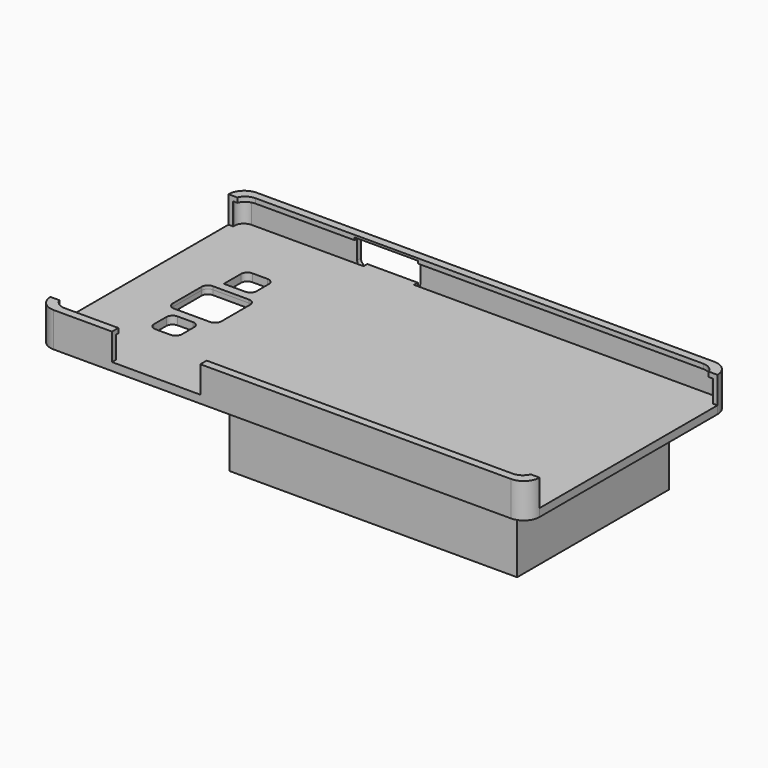
from build123d import *

# Parameters (mm, degrees)
F0_W      = 155
F0_H      = 80.5
F1_DEPTH  = 9.5
F2_T      = -1.5
F3_W      = 155
F3_H      = 80.5
F3_W_2    = 152
F3_H_2    = 77.5
F3_W_3    = 150
F3_H_3    = 75.5
F4_DEPTH  = 1.5
F5_W      = 20
F5_H      = 8.7980394721
F6_DEPTH  = 2.501
F7_W      = 8.8
F7_H      = 4.4
F7_W_2    = 15.4
F7_H_2    = 7.7
F8_DEPTH  = 1.5
F9_R      = 2
F10_R     = 5
F11_R     = 3
F12_F1_R  = 4
F12_F2_R  = 4
F12_F3_R  = 4
F12_F4_R  = 4
F13_W     = 70.5
F13_H     = 9.5
F14_DEPTH = 2.7929007565
F15_W     = 70.5
F15_H     = 9.5
F16_DEPTH = 2.7929007565
F17_W     = 28
F17_H     = 9.5
F18_DEPTH = 2.501
F19_DEPTH = 1
F20_W     = 91.1511071026
F20_H     = 60.2068249136
F21_DEPTH = 22
F22_W     = 56.2
F22_H     = 20
F23_DEPTH = 91


with BuildPart() as f1:
    # F0 (on Top) → F1 (new body)
    with BuildSketch(Plane.XY):
        with Locations((77.5, 40.25)):
            Rectangle(F0_W, F0_H)
    extrude(amount=F1_DEPTH)

    # F2
    f2_openings = [f1.faces().sort_by_distance(p)[0] for p in [
        (77.5, 40.25, 9.5),
    ]]
    offset(amount=F2_T, openings=f2_openings)

    # F3 (on face) → F4 (join)
    with BuildSketch(Plane.XY.offset(9.5)):
        with Locations((77.5, 40.25)):
            Rectangle(F3_W, F3_H)
        with Locations((77.5, 40.25)):
            Rectangle(F3_W_2, F3_H_2, mode=Mode.SUBTRACT)
        with Locations((77.5, 40.25)):
            Rectangle(F3_W_2, F3_H_2)
        with Locations((77.5, 40.25)):
            Rectangle(F3_W_3, F3_H_3, mode=Mode.SUBTRACT)
    extrude(amount=F4_DEPTH)

    # F5 (on face) → F6 (cut, through all)
    with BuildSketch(Plane(origin=(0, 80.5, 0), x_dir=(-1, 0, 0), z_dir=(0, 1, 0))):
        with Locations((-48, 5.8990197361)):
            Rectangle(F5_W, F5_H)
    extrude(amount=-F6_DEPTH, mode=Mode.SUBTRACT)

    # F7 (on face) → F8 (cut, through all)
    with BuildSketch(Plane(origin=(0, 0, 0), x_dir=(1, 0, 0), z_dir=(0, 0, -1))):
        with Locations((23.3, -27.05)):
            Rectangle(F7_W, F7_H)
        with Locations((23.3, -22.65)):
            Rectangle(F7_W, F7_H)
        with Locations((23.3, -35.8)):
            Rectangle(F7_W_2, F7_H_2)
        with Locations((23.3, -43.5)):
            Rectangle(F7_W_2, F7_H_2)
        with Locations((23.3, -52.25)):
            Rectangle(F7_W, F7_H)
        with Locations((23.3, -56.65)):
            Rectangle(F7_W, F7_H)
    extrude(amount=-F8_DEPTH, mode=Mode.SUBTRACT)

    # F9
    f9_edges = [f1.edges().sort_by_distance(p)[0] for p in [
        (18.9, 29.25, 0.75),
        (15.6, 47.35, 0.75),
        (18.9, 58.85, 0.75),
        (18.9, 20.45, 0.75),
        (15.6, 31.95, 0.75),
        (27.7, 50.05, 0.75),
        (31, 31.95, 0.75),
        (27.7, 20.45, 0.75),
        (27.7, 29.25, 0.75),
        (31, 47.35, 0.75),
        (27.7, 58.85, 0.75),
        (58, 79.75, 1.5),
        (38, 79.75, 1.5),
    ]]
    fillet(f9_edges, radius=F9_R)

    # F10
    f10_edges = [f1.edges().sort_by_distance(p)[0] for p in [
        (0, 0, 5.5),
        (0, 80.5, 5.5),
        (155, 0, 5.5),
        (155, 80.5, 5.5),
    ]]
    fillet(f10_edges, radius=F10_R)

    # F11
    f11_edges = [f1.edges().sort_by_distance(p)[0] for p in [
        (1.5, 79, 5.5),
        (1.5, 1.5, 5.5),
        (153.5, 79, 5.5),
        (153.5, 1.5, 5.5),
    ]]
    fillet(f11_edges, radius=F11_R)

    # F12: fillet of radius 4 on 4 edges, made by hand

    # F12_f1
    f12_f1_edges = [f1.edges().sort_by_distance(p)[0] for p in [
        (152.5, 78, 10.25),
    ]]
    fillet(f12_f1_edges, radius=F12_F1_R)

    # F12_f2
    f12_f2_edges = [f1.edges().sort_by_distance(p)[0] for p in [
        (2.5, 78, 10.25),
    ]]
    fillet(f12_f2_edges, radius=F12_F2_R)

    # F12_f3
    f12_f3_edges = [f1.edges().sort_by_distance(p)[0] for p in [
        (152.5, 2.5, 10.25),
    ]]
    fillet(f12_f3_edges, radius=F12_F3_R)

    # F12_f4
    f12_f4_edges = [f1.edges().sort_by_distance(p)[0] for p in [
        (2.5, 2.5, 10.25),
    ]]
    fillet(f12_f4_edges, radius=F12_F4_R)

    # F13 (on face) → F14 (cut, through all)
    with BuildSketch(Plane(origin=(0, 0, 0), x_dir=(0, -1, 0), z_dir=(-1, 0, 0))):
        with Locations((-40.25, 6.25)):
            Rectangle(F13_W, F13_H)
    extrude(amount=-F14_DEPTH, mode=Mode.SUBTRACT)

    # F15 (on face) → F16 (cut, through all)
    with BuildSketch(Plane.YZ.offset(155)):
        with Locations((40.25, 6.25)):
            Rectangle(F15_W, F15_H)
    extrude(amount=-F16_DEPTH, mode=Mode.SUBTRACT)

    # F17 (on face) → F18 (cut, through all)
    with BuildSketch(Plane.XZ):
        with Locations((37.5, 6.25)):
            Rectangle(F17_W, F17_H)
    extrude(amount=-F18_DEPTH, mode=Mode.SUBTRACT)

    # F19 (add): a face of the model
    f19_faces = [f1.faces().sort_by_distance(p)[0] for p in [
        (79.0729751372, 40.2079373473, 1.5),
    ]]
    extrude(f19_faces, amount=F19_DEPTH)

    # F20 (on face) → F21 (join)
    with BuildSketch(Plane(origin=(0, 0, 0), x_dir=(1, 0, 0), z_dir=(0, 0, -1))):
        with Locations((98.8614168018, -39.4122553989)):
            Rectangle(F20_W, F20_H)
    extrude(amount=F21_DEPTH)

    # F22 (on face) → F23 (cut)
    with BuildSketch(Plane(origin=(53.2858632505, 0, 0), x_dir=(0, -1, 0), z_dir=(-1, 0, 0))):
        with Locations((-39.4156678557, -10)):
            Rectangle(F22_W, F22_H)
    extrude(amount=-F23_DEPTH, mode=Mode.SUBTRACT)


solid = f1.part
